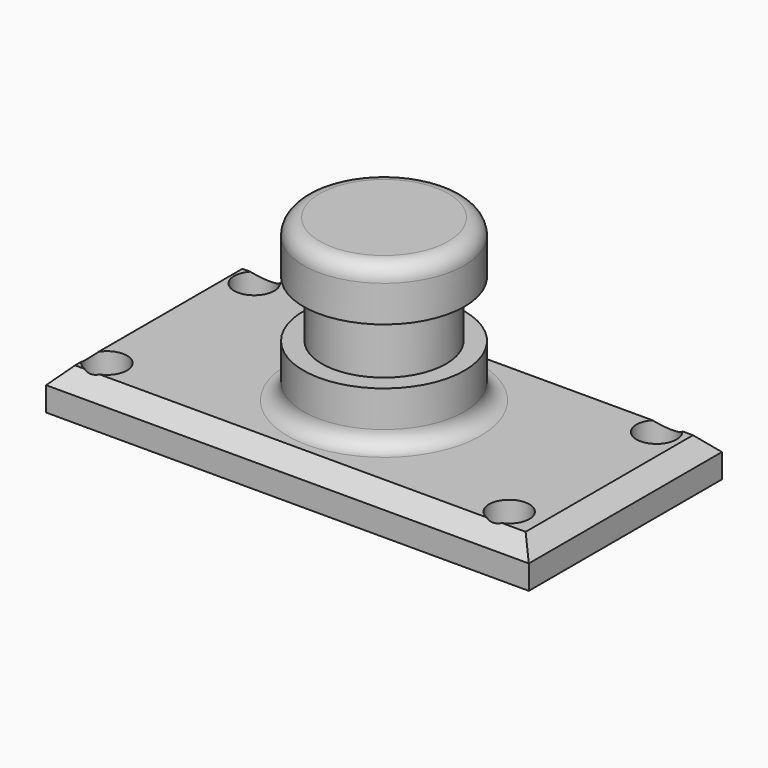
from build123d import *

# Parameters (mm, degrees)
F0_W        = 152.4
F0_H        = 76.2
F1_DEPTH    = 12.7
F2_R        = 6.35
F3_DEPTH    = 12.701
F4_W        = 25.4
F4_H        = 50.8
F6_W        = 11.3594501876
F6_H        = 17.78
F8_R        = 5.08
F9_T1_DEPTH = 102.3282991577
F9_T3_DEPTH = 178.5282991577


# Not quite as in the source:
# - a fillet or chamfer that OpenCascade refuses, or shapes differently, is made with other operations: its cross-section is extruded or revolved along the edge and cut away or added


with BuildPart() as f1:
    # F0 (on Top) → F1 (new body)
    with BuildSketch(Plane.XY):
        Rectangle(F0_W, F0_H)
    extrude(amount=F1_DEPTH)

    # F2 (on face) → F3 (cut, through all)
    with BuildSketch(Plane.XY.offset(12.7)):
        with Locations((-63.9521719884, 28.7373781539)):
            Circle(F2_R)
        with Locations((-65.762154874, -27.1426218461)):
            Circle(F2_R)
        with Locations((63.0478280116, 28.7373781539)):
            Circle(F2_R)
        with Locations((61.237845126, -27.1426218461)):
            Circle(F2_R)
    extrude(amount=-F3_DEPTH, mode=Mode.SUBTRACT)

    # F4 (on Front) → F5 (revolve)
    with BuildSketch(Plane.XZ):
        with Locations((12.7, 38.1)):
            Rectangle(F4_W, F4_H)
    revolve(axis=Axis((0, 0, 38.1), (0, 0, 1)))

    # F6 (on Front) → F7 (revolve, cut)
    with BuildSketch(Plane.XZ):
        with Locations((25.2974471077, 38.0985615775)):
            Rectangle(F6_W, F6_H)
    revolve(axis=Axis((0, 0, 12.7), (0, 0, 1)), mode=Mode.SUBTRACT)

    # F8
    f8_edges = [f1.edges().sort_by_distance(p)[0] for p in [
        (-25.4, 0, 63.5),
        (-25.4, 0, 12.7),
    ]]
    fillet(f8_edges, radius=F8_R)

    # F9: chamfer of 5.08 on 4 edges, made by hand

    # F9_s2 → F9_t1 (cut)
    with BuildSketch(Plane.XZ.offset(-51.1641495789)):
        Polygon((71.12, 12.7), (76.2, 7.62), (76.2, 12.7), align=None)
        Polygon((-71.12, 12.7), (-76.2, 7.62), (-76.2, 12.7), align=None)
    extrude(amount=F9_T1_DEPTH, mode=Mode.SUBTRACT)

    # F9_s4 → F9_t3 (cut)
    with BuildSketch(Plane.YZ.offset(-89.2641495789)):
        Polygon((33.02, 12.7), (38.1, 7.62), (38.1, 12.7), align=None)
        Polygon((-33.02, 12.7), (-38.1, 7.62), (-38.1, 12.7), align=None)
    extrude(amount=F9_T3_DEPTH, mode=Mode.SUBTRACT)


solid = f1.part
